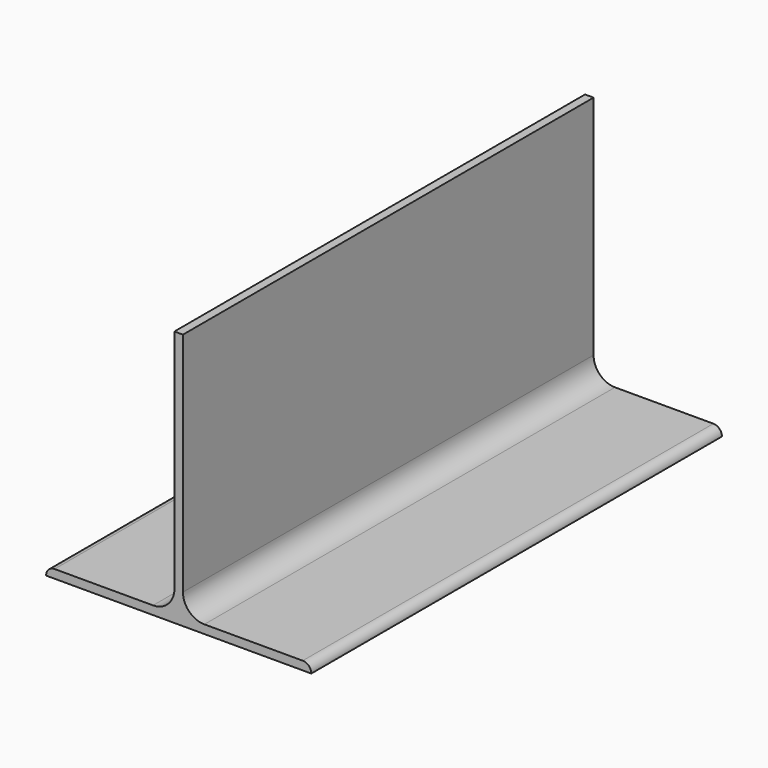
from build123d import *

# Parameters (mm, degrees)
F1_DEPTH = 120
F2_R     = 5
F3_R     = 1.99999


# Not quite as in the source:
# - a fillet or chamfer is up to 0.001 mm smaller than in the source, because OpenCascade refuses the exact size


with BuildPart() as f1:
    # F0 (on Front) → F1 (new body)
    with BuildSketch(Plane.XZ):
        Polygon((1, 60), (0, 60), (-1, 60), (-1, 2), (-31, 2), (-31, 0), (0, 0), (31, 0), (31, 2), (1, 2), align=None)
    extrude(amount=F1_DEPTH)

    # F2
    f2_edges = [f1.edges().sort_by_distance(p)[0] for p in [
        (-1, -60, 2),
        (1, -60, 2),
    ]]
    fillet(f2_edges, radius=F2_R)

    # F3 (radius 2 in the source; OpenCascade refuses exactly that, so slightly less here)
    f3_edges = [f1.edges().sort_by_distance(p)[0] for p in [
        (31, -60, 2),
        (-31, -60, 2),
    ]]
    fillet(f3_edges, radius=F3_R)


solid = f1.part
